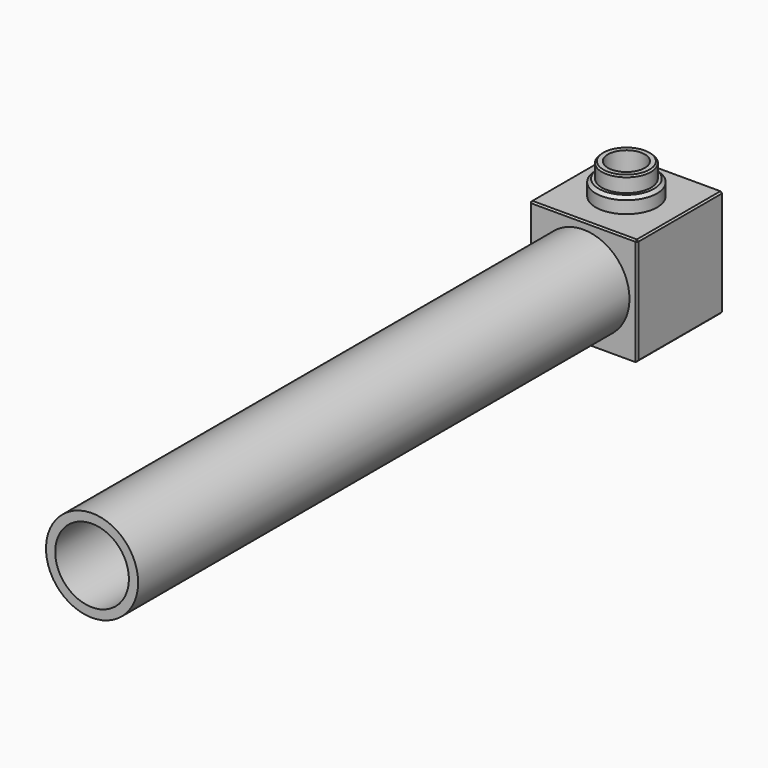
from build123d import *

# Parameters (mm, degrees)
F0_W      = 35
F0_H      = 35
F1_DEPTH  = 35
F2_R      = 15
F2_R_2    = 12
F3_DEPTH  = 200
F4_R      = 10
F5_DEPTH  = 5
F6_R      = 8
F7_DEPTH  = 5
F8_SIZE   = 1
F9_SIZE   = 0.5
F10_R     = 6
F11_DEPTH = 35
F12_SIZE  = 0.5


# Not quite as in the source:
# - a feature names something its author has since deleted; it is built from what else it names


with BuildPart() as f1:
    # F0 (on Front) → F1 (new body)
    with BuildSketch(Plane.XZ):
        Rectangle(F0_W, F0_H)
    extrude(amount=F1_DEPTH)

    # F2 (on face) → F3 (join)
    with BuildSketch(Plane.XZ.offset(35)):
        Circle(F2_R)
        Circle(F2_R_2, mode=Mode.SUBTRACT)
    extrude(amount=F3_DEPTH)

    # F4 (on face) → F5 (join)
    with BuildSketch(Plane.XY.offset(17.5)):
        with Locations((0, -17.5)):
            Circle(F4_R)
    extrude(amount=F5_DEPTH)

    # F6 (on face) → F7 (join)
    with BuildSketch(Plane.XY.offset(22.5)):
        with Locations((0, -17.5)):
            Circle(F6_R)
    extrude(amount=F7_DEPTH)

    # F8
    f8_edges = [f1.edges().sort_by_distance(p)[0] for p in [
        (-10, -17.5, 22.5),
    ]]
    chamfer(f8_edges, length=F8_SIZE)

    # F9
    f9_edges = [f1.edges().sort_by_distance(p)[0] for p in [
        (-8, -17.5, 27.5),
    ]]
    chamfer(f9_edges, length=F9_SIZE)

    # F10 (on face) → F11 (cut)
    with BuildSketch(Plane.XY.offset(27.5)):
        with Locations((0, -17.5)):
            Circle(F10_R)
    extrude(amount=-F11_DEPTH, mode=Mode.SUBTRACT)

    # F12
    f12_edges = [f1.edges().sort_by_distance(p)[0] for p in [
        (0, -35, 17.5),
        (-17.5, -17.5, 17.5),
        (17.5, -17.5, 17.5),
        (0, 0, 17.5),
        (17.5, 0, 0),
        (17.5, -35, 0),
        (17.5, -17.5, -17.5),
        (0, 0, -17.5),
        (-17.5, -35, 0),
        (-17.5, -17.5, -17.5),
        (-17.5, 0, 0),
    ]]
    chamfer(f12_edges, length=F12_SIZE)


solid = f1.part
